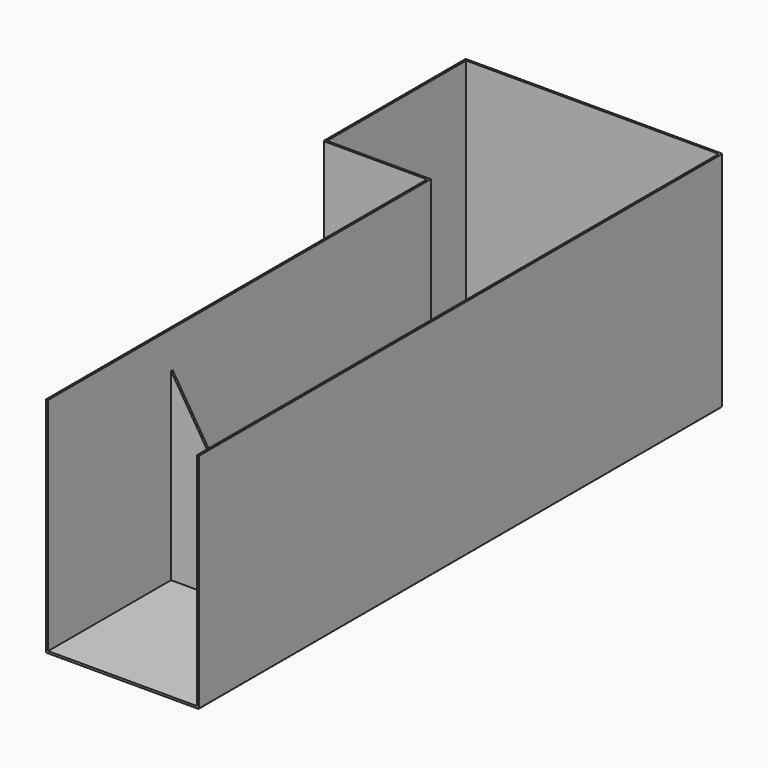
from build123d import *

# Parameters (mm, degrees)
F1_DEPTH  = 426
F3_DEPTH  = 4
F4_R      = 2
F7_DEPTH  = 4
F10_DEPTH = 4


# Not quite as in the source:
# - a feature names something its author has since deleted; it is built from what else it names


with BuildPart() as f1:
    # F0 (on Top) → F1 (new body)
    with BuildSketch(Plane.XY):
        Polygon((495, 0), (0, 0), (0, -343), (200, -343), (200, -1261), (204, -1261), (204, -339), (4, -339), (4, -4), (491, -4), (491, -1261), (495, -1261), align=None)
    extrude(amount=F1_DEPTH)

    # F2 (on Top) → F3 (join)
    with BuildSketch(Plane.XY):
        Polygon((0, -343), (200, -343), (200, -1261), (495, -1261), (495, 0), (0, 0), align=None)
    extrude(amount=-F3_DEPTH)

    # F4
    f4_edges = [f1.edges().sort_by_distance(p)[0] for p in [
        (100, -343, -4),
        (0, -171.5, -4),
        (247.5, 0, -4),
        (200, -343, 211),
        (0, -343, 211),
        (0, 0, 211),
        (495, 0, 211),
        (200, -802, -4),
        (495, -630.5, -4),
    ]]
    fillet(f4_edges, radius=F4_R)

    # F6 (on offset) → F7 (join)
    with BuildSketch(Plane.XZ.offset(961)):
        Polygon((204, 355), (204, 0), (426, 0), align=None)
    extrude(amount=F7_DEPTH)

    # F9 (on offset) → F10 (join)
    with BuildSketch(Plane.XZ.offset(365)):
        Polygon((269, 0), (491, 0), (491, 355), align=None)
    extrude(amount=F10_DEPTH)


solid = f1.part
